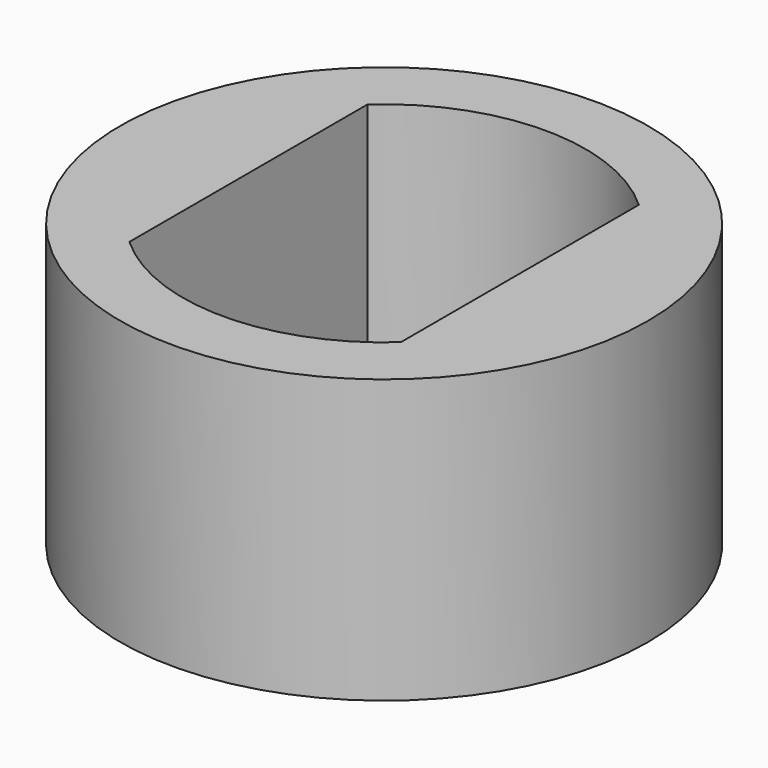
from build123d import *

# Parameters (mm, degrees)
F0_R     = 4.445
F1_DEPTH = 4.7625


# Not quite as in the source:
# - a length typed as a fraction of an inch, garbled in the dataset ("3 / 203.2 mm" for 3/8 in), is restored


with BuildPart() as f1:
    # F0 (on Top) → F1 (new body)
    with BuildSketch(Plane.XY):
        Circle(F0_R)
        with BuildLine():
            ThreePointArc((2.286, 2.5044773527), (3.1024023119, 1.3686864889), (3.3909, 0))
            ThreePointArc((3.3909, 0), (3.1024023119, -1.3686864889), (2.286, -2.5044773527))
            ThreePointArc((2.286, -2.5044773527), (0, -3.3909), (-2.286, -2.5044773527))
            ThreePointArc((-2.286, -2.5044773527), (-3.3909, 0), (-2.286, 2.5044773527))
            ThreePointArc((-2.286, 2.5044773527), (0, 3.3909), (2.286, 2.5044773527))
        make_face(mode=Mode.SUBTRACT)
        with BuildLine():
            Line((-2.286, -2.5044773527), (-2.286, 2.5044773527))
            ThreePointArc((-2.286, 2.5044773527), (-3.3909, 0), (-2.286, -2.5044773527))
        make_face()
        with BuildLine():
            ThreePointArc((2.286, -2.5044773527), (3.1024023119, -1.3686864889), (3.3909, 0))
            ThreePointArc((3.3909, 0), (3.1024023119, 1.3686864889), (2.286, 2.5044773527))
            Line((2.286, 2.5044773527), (2.286, -2.5044773527))
        make_face()
    extrude(amount=F1_DEPTH)


solid = f1.part
